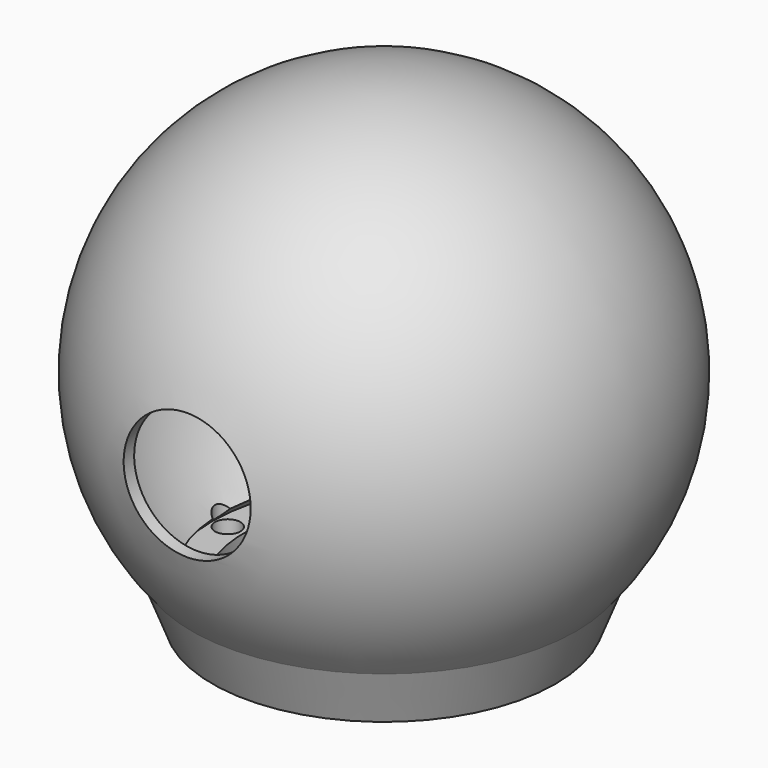
from build123d import *

# Parameters (mm, degrees)
F0_W     = 6.35
F0_H     = 6.35
F2_D     = 25.4
F2_DEPTH = 50.801
F4_D     = 5.08
F4_DEPTH = 43.832140591
F6_D     = 5.08
F6_DEPTH = 43.832140591
F7_D     = 5.08
F7_DEPTH = 43.832140591


with BuildPart() as f1:
    # F0 (on Front) → F1 (revolve)
    with BuildSketch(Plane.XZ):
        with BuildLine():
            ThreePointArc((38.401894824, -33.2555931225), (46.2061907682, 21.1099013425), (0, 50.8))
            Line((0, 50.8), (0, 48.26))
            ThreePointArc((0, 48.26), (44.9856946855, 17.4732616779), (32.5755, -35.6070835614))
            Line((32.5755, -35.6070835614), (34.29, -37.481140591))
            ThreePointArc((34.29, -37.481140591), (36.407302923, -35.4280721162), (38.401894824, -33.2555931225))
        make_face()
        with Locations((31.115, -40.656140591)):
            Rectangle(F0_W, F0_H)
        with BuildLine():
            Line((34.29, -43.831140591), (38.401894824, -33.2555931225))
            ThreePointArc((38.401894824, -33.2555931225), (36.407302923, -35.4280721162), (34.29, -37.481140591))
            Line((34.29, -37.481140591), (34.29, -43.831140591))
        make_face()
    revolve(axis=Axis((0, 0, 49.53), (0, 0, 1)))

    # F2 (through all, one way)
    with BuildSketch(Plane(origin=(0, 0, 0), x_dir=(1, 0, 0), z_dir=(0, 1, 0))):
        with Locations((0, 0)):
            Circle(F2_D / 2)
    extrude(amount=-F2_DEPTH, mode=Mode.SUBTRACT)

    # F4 (through all, one way)
    with BuildSketch(Plane.XY):
        with Locations((-31.242, 0)):
            Circle(F4_D / 2)
    extrude(amount=-F4_DEPTH, mode=Mode.SUBTRACT)

    # F6 (through all, one way)
    with BuildSketch(Plane.XY):
        with Locations((0, -30.988)):
            Circle(F6_D / 2)
    extrude(amount=-F6_DEPTH, mode=Mode.SUBTRACT)

    # F7 (through all, one way)
    with BuildSketch(Plane.XY):
        with Locations((0, 31.242), (31.242, 0)):
            Circle(F7_D / 2)
    extrude(amount=-F7_DEPTH, mode=Mode.SUBTRACT)


solid = f1.part
